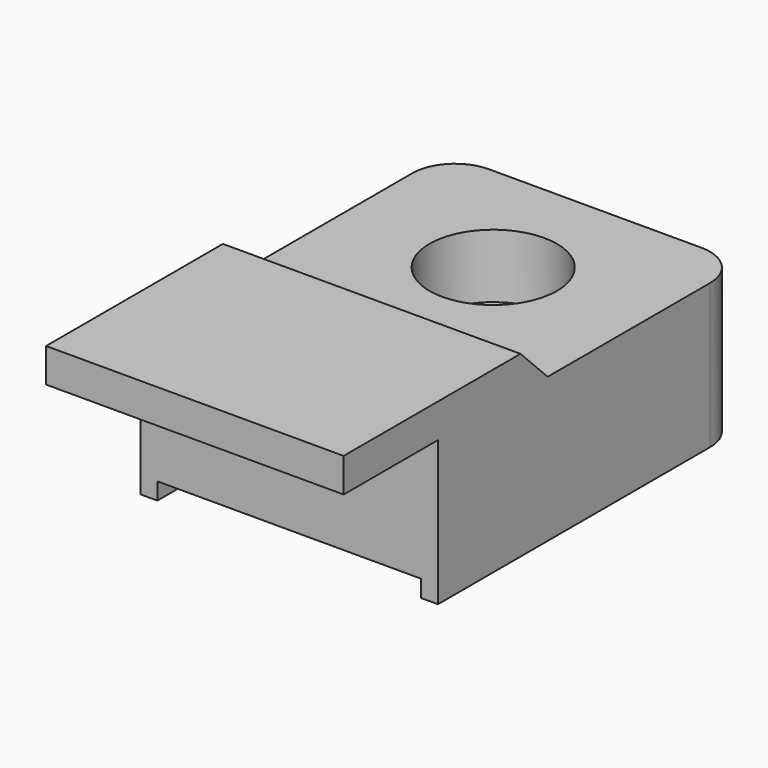
from build123d import *

# Parameters (mm, degrees)
F0_W      = 35
F0_H      = 45
F1_DEPTH  = 15
F2_W      = 2
F2_H      = 45
F3_DEPTH  = 2
F4_W      = 35
F4_H      = 13.8643281162
F4_H_2    = 16.1356718838
F5_DEPTH  = 4
F6_SIZE   = 3.99999
F7_R      = 3.25
F8_DEPTH  = 15
F9_R      = 5
F10_R     = 7.5
F10_R_2   = 3.25
F11_DEPTH = 7.5


# Not quite as in the source:
# - a fillet or chamfer is up to 0.001 mm smaller than in the source, because OpenCascade refuses the exact size


with BuildPart() as f1:
    # F0 (on Top) → F1 (new body)
    with BuildSketch(Plane.XY):
        Rectangle(F0_W, F0_H)
    extrude(amount=F1_DEPTH)

    # F2 (on face) → F3 (join)
    with BuildSketch(Plane(origin=(0, 0, 0), x_dir=(1, 0, 0), z_dir=(0, 0, -1))):
        with Locations((-16.5, 0)):
            Rectangle(F2_W, F2_H)
        with Locations((16.5, 0)):
            Rectangle(F2_W, F2_H)
    extrude(amount=F3_DEPTH)

    # F4 (on face) → F5 (join)
    with BuildSketch(Plane.XY.offset(15)):
        with Locations((0, -29.4321640581)):
            Rectangle(F4_W, F4_H)
        with Locations((0, -14.4321640581)):
            Rectangle(F4_W, F4_H_2)
    extrude(amount=F5_DEPTH)

    # F6 (size 4 in the source; OpenCascade refuses exactly that, so slightly less here)
    f6_edges = [f1.edges().sort_by_distance(p)[0] for p in [
        (0, -6.364328, 19),
    ]]
    chamfer(f6_edges, length=F6_SIZE)

    # F7 (on face) → F8 (cut, through all)
    with BuildSketch(Plane.XY.offset(15)):
        with Locations((0, 7.5)):
            Circle(F7_R)
    extrude(amount=-F8_DEPTH, mode=Mode.SUBTRACT)

    # F9
    f9_edges = [f1.edges().sort_by_distance(p)[0] for p in [
        (-17.5, 22.5, 6.5),
        (17.5, 22.5, 6.5),
    ]]
    fillet(f9_edges, radius=F9_R)

    # F10 (on face) → F11 (cut)
    with BuildSketch(Plane.XY.offset(15)):
        with Locations((0, 7.5)):
            Circle(F10_R)
        with Locations((0, 7.5)):
            Circle(F10_R_2, mode=Mode.SUBTRACT)
    extrude(amount=-F11_DEPTH, mode=Mode.SUBTRACT)


solid = f1.part
